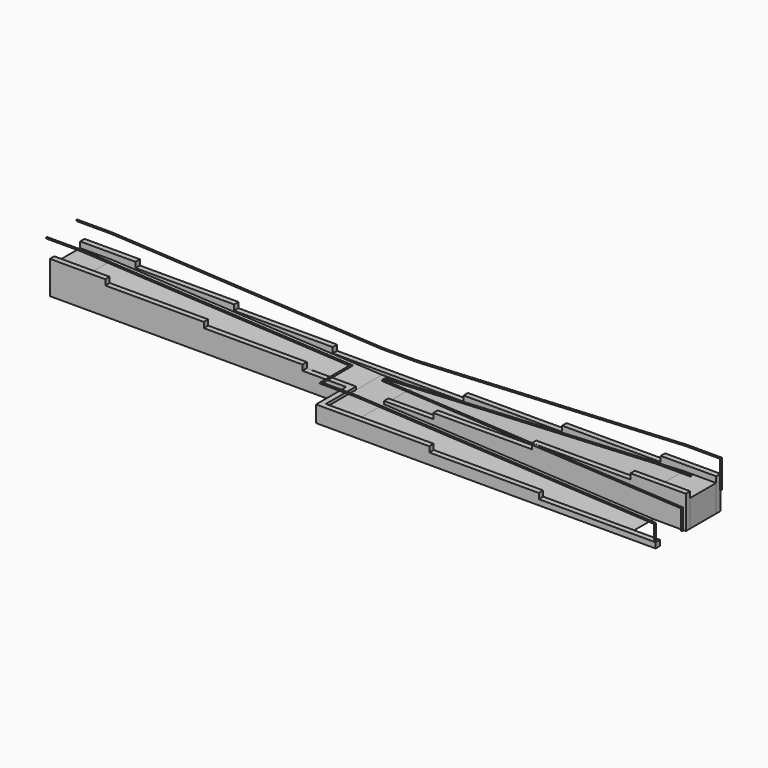
from build123d import *

# Parameters (mm, degrees)
F1_DEPTH  = 1200
F2_DEPTH  = 1403.2
F3_W      = 11200
F3_H      = 203.2
F4_DEPTH  = 1000.001
F7_DEPTH  = 203.2
F9_DEPTH  = 203.2
F11_DEPTH = 203.2
F13_DEPTH = 203.2
F24_R     = 25.4
F26_R     = 25.4
F29_R     = 25.4


# Not quite as in the source:
# - the program builds the solid bodies; features that only make, move or delete a surface that nothing else refers to are left out


with BuildPart() as f1:
    # F0 (on Front) → F1 (new body)
    with BuildSketch(Plane.XZ):
        Polygon((-10000, 0), (0, 0), (-10000, 500), (-11200, 500), (-11200, 0), align=None)
    extrude(amount=F1_DEPTH)

    # F0 (on Front) → F2 (join)
    with BuildSketch(Plane.XZ):
        Polygon((-10000, 500), (0, 0), (1200, 0), (1200, 1000), (0, 1000), align=None)
        Polygon((-10000, 0), (0, 0), (-10000, 500), (-11200, 500), (-11200, 0), align=None)
        Polygon((-21200, 0), (-11200, 0), (-11200, 500), (-21200, 1000), (-22400, 1000), (-22400, 0), align=None)
    extrude(amount=-F2_DEPTH)

    # F3 (on Top) → F4 (cut, through all)
    with BuildSketch(Plane.XY):
        with Locations((-4400, 101.6)):
            Rectangle(F3_W, F3_H)
        with Locations((-16800, 101.6)):
            Rectangle(F3_W, F3_H)
    extrude(amount=F4_DEPTH, mode=Mode.SUBTRACT)


with BuildPart() as f7:
    # F6 (on face) → F7 (new body)
    with BuildSketch(Plane.XZ.offset(-203.2)):
        Polygon((-10000, 609.6), (-10000, 0), (1200, 0), (1200, 1219.2), (-856, 1219.2), (-856, 1016), (-4513.6, 1016), (-4513.6, 812.8), (-8171.2, 812.8), (-8171.2, 609.6), align=None)
    extrude(amount=F7_DEPTH)


with BuildPart() as f7b:
    # F6 (on face) → F7, piece 2 (new body)
    with BuildSketch(Plane.XZ.offset(-203.2)):
        Polygon((-16688.2814086914, 1016), (-20345.8814086914, 1016), (-20345.8814086914, 1219.2), (-22401.8814086914, 1219.2), (-22401.8814086914, 0), (-11201.8814086914, 0), (-11201.8814086914, 609.6), (-13030.6814086914, 609.6), (-13030.6814086914, 812.8), (-16688.2814086914, 812.8), align=None)
    extrude(amount=F7_DEPTH)

    # F10 (on face) → F11 (join)
    with BuildSketch(Plane(origin=(-11200, 0, 0), x_dir=(0, -1, 0), z_dir=(-1, 0, 0))):
        Polygon((0, 609.6), (0, 0), (1200, 0), (1403.2, 0), (1403.2, 609.6), (1200, 609.6), align=None)
    extrude(amount=F11_DEPTH)

    # F12 (on face) → F13 (join)
    with BuildSketch(Plane.XZ.offset(1200)):
        Polygon((-11200, 609.6), (-11200, 500), (-11200, 0), (1200, 0), (1200, 203.2), (928, 203.2), (-3136, 203.2), (-3136, 406.4), (-7200, 406.4), (-7200, 609.6), align=None)
    extrude(amount=F13_DEPTH)


with BuildPart() as f9:
    # F8 (on face) → F9 (new body)
    with BuildSketch(Plane(origin=(0, 1403.2, 0), x_dir=(-1, 0, 0), z_dir=(0, 1, 0))):
        Polygon((11200, 609.6), (10000, 609.6), (8171.2, 609.6), (8171.2, 812.8), (4513.6, 812.8), (4513.6, 1016), (856, 1016), (856, 1219.2), (-1200, 1219.2), (-1200, 0), (10000, 0), (11200, 0), (22400, 0), (22400, 1219.2), (20344, 1219.2), (20344, 1016), (16686.4, 1016), (16686.4, 812.8), (13028.8, 812.8), (13028.8, 609.6), align=None)
    extrude(amount=F9_DEPTH)


with BuildPart() as f25:
    # F25: sweep along a path in F15, F18, F21
    with BuildLine(Plane.XZ.offset(1301.6)) as f25_path:
        Line((1098.4, 0), (1098.4, 745.08))
        Line((1098.4, 745.08), (-10000, 1300))
    with BuildLine(Plane.XY.offset(1300)) as f25_path_2:
        Line((-10000, -1301.6), (-11301.6, -1301.6))
        Line((-11301.6, -1301.6), (-11301.6, 101.6))
    with BuildLine(Plane.XZ.offset(-101.6)) as f25_path_3:
        Line((-11301.6, 1300), (-21301.6, 1800))
        Line((-21301.6, 1800), (-22603.2, 1800))
    # F24 (on Top) → F25 (sweep)
    with BuildSketch(Plane.XY):
        with Locations((1098.4, -1301.6)):
            Circle(F24_R)
    sweep(path=f25_path.line + f25_path_2.line + f25_path_3.line, transition=Transition.RIGHT)


with BuildPart() as f27:
    # F27: sweep along a path in F23, F18, F21
    with BuildLine(Plane.XZ.offset(50.8)) as f27_path:
        Line((1098.4, 0), (1098.4, 745.08))
        Line((1098.4, 745.08), (-10000, 1300))
    with BuildLine(Plane.XY.offset(1300)) as f27_path_2:
        Line((-10000, 101.6), (-10000, -50.8))
    with BuildLine(Plane.XZ.offset(-101.6)) as f27_path_3:
        Line((-10000, 1300), (0, 1800))
        Line((0, 1800), (1301.6, 1800))
    # F26 (on Top) → F27 (sweep)
    with BuildSketch(Plane.XY):
        with Locations((1098.4, -50.8)):
            Circle(F26_R)
    sweep(path=f27_path.line + f27_path_2.line + f27_path_3.line, transition=Transition.RIGHT)


with BuildPart() as f30:
    # F30: sweep along a path in F30_path
    with BuildLine(Plane(origin=(1301.6, 1504.8, 1800), x_dir=(0, 0, 1), z_dir=(0, -1, 0))) as f30_path:
        Line((-1026.9801497459, 0), (0, 0))
        Line((0, 0), (0, 1301.6))
        Line((0, 1301.6), (-500, 11301.6))
        Line((-500, 11301.6), (-500, 12603.2))
        Line((-500, 12603.2), (0, 22603.2))
        Line((0, 22603.2), (0, 23904.8))
    # F29 (on plane+point) → F30 (sweep)
    with BuildSketch(Plane.XY.offset(773.0198502541)):
        with Locations((1301.6, 1504.8)):
            Circle(F29_R)
    sweep(path=f30_path.line, transition=Transition.RIGHT)


solid = Compound([f1.part, f7.part, f7b.part, f9.part, f25.part, f27.part, f30.part])
